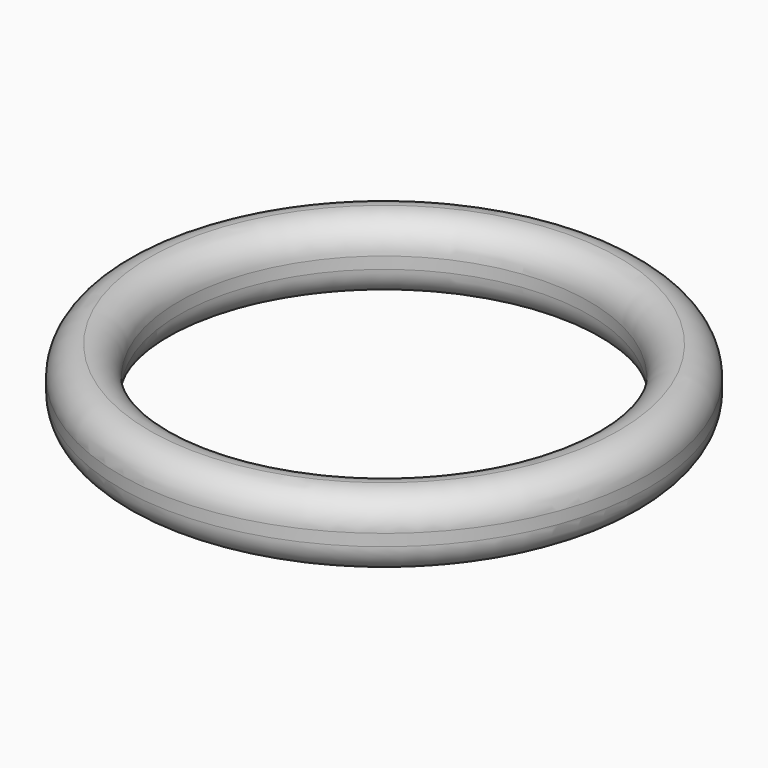
from build123d import *

# Parameters (mm, degrees)
F0_R     = 4.5
F0_R_2   = 3.5
F1_DEPTH = 1.2
F2_R     = 0.49999


# Not quite as in the source:
# - a fillet or chamfer is up to 0.001 mm smaller than in the source, because OpenCascade refuses the exact size


with BuildPart() as f1:
    # F0 (on Top) → F1 (new body)
    with BuildSketch(Plane.XY):
        Circle(F0_R)
        Circle(F0_R_2, mode=Mode.SUBTRACT)
    extrude(amount=F1_DEPTH)

    # F2 (radius 0.5 in the source; OpenCascade refuses exactly that, so slightly less here)
    f2_edges = [f1.edges().sort_by_distance(p)[0] for p in [
        (-4.5, 0, 1.2),
        (-4.5, 0, 0),
        (-3.5, 0, 0),
        (-3.5, 0, 1.2),
    ]]
    fillet(f2_edges, radius=F2_R)


solid = f1.part
